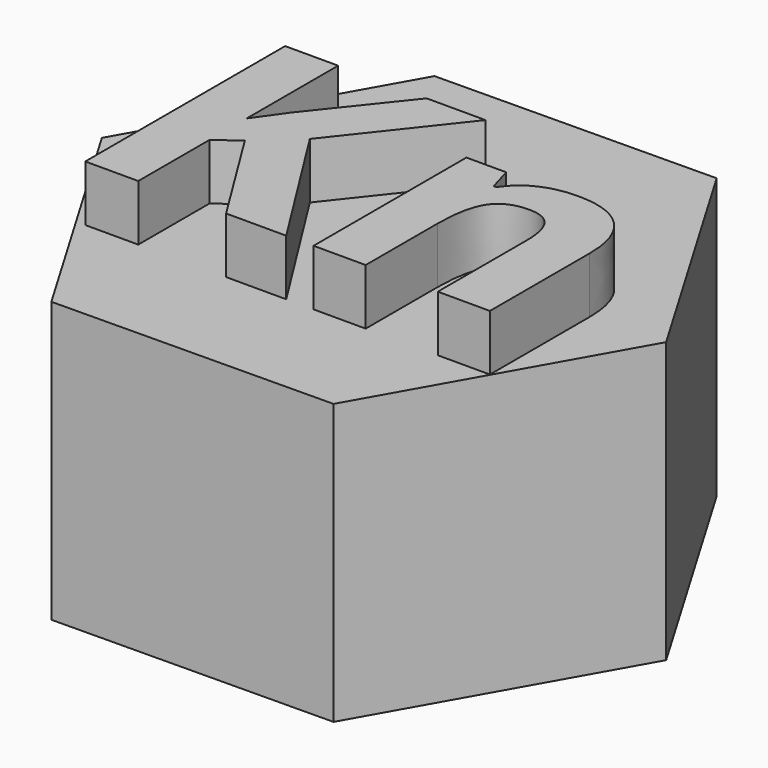
from build123d import *

# Parameters (mm, degrees)
F1_DEPTH     = 12.7
F2_TEXT_SIZE = 15.875001231
F3_DEPTH     = 2.54


# Not quite as in the source:
# - Text() gives the source's letters only with a copy of the font that has no kerning and outlines rounded to 1/6400 em; it was checked with that copy


with BuildPart() as f1:
    # F0 (on Top) → F1 (new body)
    with BuildSketch(Plane.XY):
        Polygon((12.6993846473, 0.1250183213), (6.2414232815, 11.0604988776), (-6.4579613658, 10.9354805563), (-12.6993846473, -0.1250183213), (-6.2414232815, -11.0604988776), (6.4579613658, -10.9354805563), align=None)
    extrude(amount=F1_DEPTH)

    # F2 (on face) → F3 (join)
    with BuildSketch(Plane.XY.offset(12.7)):
        with Locations((-10.4055672131, -5.7150004432)):
            Text('Kn', F2_TEXT_SIZE, font='Open Sans', font_style=FontStyle.BOLD, text_align=(TextAlign.LEFT, TextAlign.BOTTOM))
    extrude(amount=F3_DEPTH)


solid = f1.part
